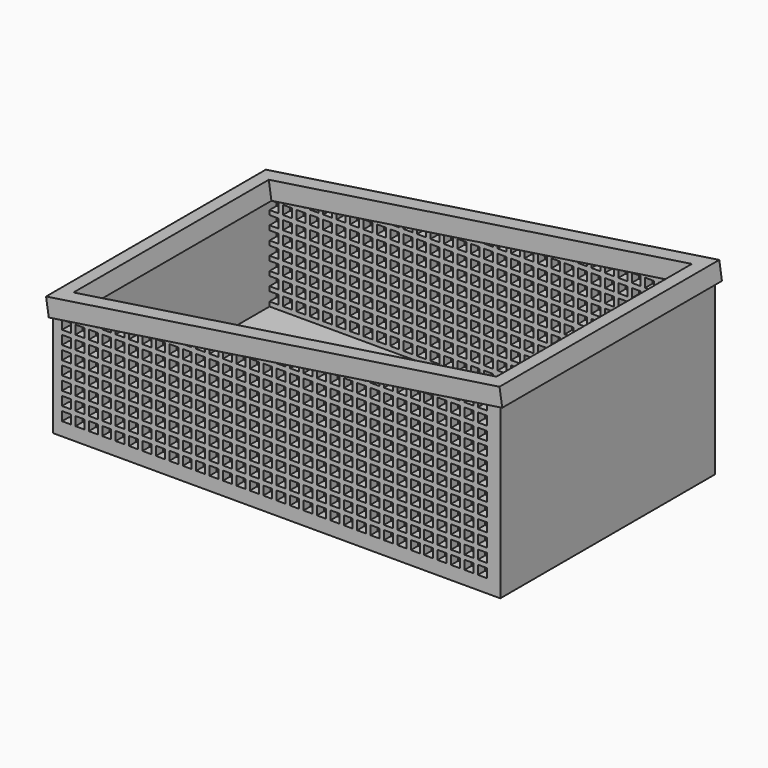
from build123d import *

# Parameters (mm, degrees)
F0_W     = 1270
F0_H     = 762
F1_DEPTH = 508
F3_W     = 1219.2
F3_H     = 711.2
F4_DEPTH = 482.6
F5_DEPTH = 762
F7_W     = 25.4
F7_H     = 25.4
F8_DEPTH = 762
F6_W     = 1302.1685366681
F6_H     = 779.9605122421
F6_W_2   = 1214.8791912068
F6_H_2   = 693.2394877579
F9_DEPTH = 25.4


with BuildPart() as f1:
    # F0 (on Top) → F1 (new body)
    with BuildSketch(Plane.XY):
        with Locations((-15.1927470725, -190.3446181417)):
            Rectangle(F0_W, F0_H)
    extrude(amount=F1_DEPTH)

    # F3 (on face) → F4 (cut)
    with BuildSketch(Plane.XY.offset(508)):
        with Locations((-15.1927470725, -190.3446181417)):
            Rectangle(F3_W, F3_H)
    extrude(amount=-F4_DEPTH, mode=Mode.SUBTRACT)

    # F2 (on face) → F5 (cut)
    with BuildSketch(Plane.XZ.offset(571.3446181417)):
        Polygon((-650.1927470725, 508), (-650.1927470725, 317.5), (619.8072529275, 508), align=None)
    extrude(amount=-F5_DEPTH, mode=Mode.SUBTRACT)

    # F7 (on face) → F8 (cut)
    with BuildSketch(Plane(origin=(0, 190.6553818583, 0), x_dir=(-1, 0, 0), z_dir=(0, 1, 0))):
        with Locations((-569.0072529275, 50.8)):
            Rectangle(F7_W, F7_H)
        with Locations((-569.0072529275, 88.9)):
            Rectangle(F7_W, F7_H)
        with Locations((-569.0072529275, 127)):
            Rectangle(F7_W, F7_H)
        with Locations((-569.0072529275, 165.1)):
            Rectangle(F7_W, F7_H)
        with Locations((-569.0072529275, 203.2)):
            Rectangle(F7_W, F7_H)
        with Locations((-569.0072529275, 241.3)):
            Rectangle(F7_W, F7_H)
        with Locations((-569.0072529275, 279.4)):
            Rectangle(F7_W, F7_H)
        with Locations((-569.0072529275, 317.5)):
            Rectangle(F7_W, F7_H)
        with Locations((-569.0072529275, 355.6)):
            Rectangle(F7_W, F7_H)
        with Locations((-530.9072529275, 50.8)):
            Rectangle(F7_W, F7_H)
        with Locations((-530.9072529275, 88.9)):
            Rectangle(F7_W, F7_H)
        with Locations((-530.9072529275, 127)):
            Rectangle(F7_W, F7_H)
        with Locations((-530.9072529275, 165.1)):
            Rectangle(F7_W, F7_H)
        with Locations((-530.9072529275, 203.2)):
            Rectangle(F7_W, F7_H)
        with Locations((-530.9072529275, 241.3)):
            Rectangle(F7_W, F7_H)
        with Locations((-530.9072529275, 279.4)):
            Rectangle(F7_W, F7_H)
        with Locations((-530.9072529275, 317.5)):
            Rectangle(F7_W, F7_H)
        with Locations((-530.9072529275, 355.6)):
            Rectangle(F7_W, F7_H)
        with Locations((-492.8072529275, 50.8)):
            Rectangle(F7_W, F7_H)
        with Locations((-492.8072529275, 88.9)):
            Rectangle(F7_W, F7_H)
        with Locations((-492.8072529275, 127)):
            Rectangle(F7_W, F7_H)
        with Locations((-492.8072529275, 165.1)):
            Rectangle(F7_W, F7_H)
        with Locations((-492.8072529275, 203.2)):
            Rectangle(F7_W, F7_H)
        with Locations((-492.8072529275, 241.3)):
            Rectangle(F7_W, F7_H)
        with Locations((-492.8072529275, 279.4)):
            Rectangle(F7_W, F7_H)
        with Locations((-492.8072529275, 317.5)):
            Rectangle(F7_W, F7_H)
        with Locations((-492.8072529275, 355.6)):
            Rectangle(F7_W, F7_H)
        with Locations((-454.7072529275, 50.8)):
            Rectangle(F7_W, F7_H)
        with Locations((-454.7072529275, 88.9)):
            Rectangle(F7_W, F7_H)
        with Locations((-454.7072529275, 127)):
            Rectangle(F7_W, F7_H)
        with Locations((-454.7072529275, 165.1)):
            Rectangle(F7_W, F7_H)
        with Locations((-454.7072529275, 203.2)):
            Rectangle(F7_W, F7_H)
        with Locations((-454.7072529275, 241.3)):
            Rectangle(F7_W, F7_H)
        with Locations((-454.7072529275, 279.4)):
            Rectangle(F7_W, F7_H)
        with Locations((-454.7072529275, 317.5)):
            Rectangle(F7_W, F7_H)
        with Locations((-454.7072529275, 355.6)):
            Rectangle(F7_W, F7_H)
        with Locations((-416.6072529275, 50.8)):
            Rectangle(F7_W, F7_H)
        with Locations((-416.6072529275, 88.9)):
            Rectangle(F7_W, F7_H)
        with Locations((-416.6072529275, 127)):
            Rectangle(F7_W, F7_H)
        with Locations((-416.6072529275, 165.1)):
            Rectangle(F7_W, F7_H)
        with Locations((-416.6072529275, 203.2)):
            Rectangle(F7_W, F7_H)
        with Locations((-416.6072529275, 241.3)):
            Rectangle(F7_W, F7_H)
        with Locations((-416.6072529275, 279.4)):
            Rectangle(F7_W, F7_H)
        with Locations((-416.6072529275, 317.5)):
            Rectangle(F7_W, F7_H)
        with Locations((-416.6072529275, 355.6)):
            Rectangle(F7_W, F7_H)
        with Locations((-378.5072529275, 50.8)):
            Rectangle(F7_W, F7_H)
        with Locations((-378.5072529275, 88.9)):
            Rectangle(F7_W, F7_H)
        with Locations((-378.5072529275, 127)):
            Rectangle(F7_W, F7_H)
        with Locations((-378.5072529275, 165.1)):
            Rectangle(F7_W, F7_H)
        with Locations((-378.5072529275, 203.2)):
            Rectangle(F7_W, F7_H)
        with Locations((-378.5072529275, 241.3)):
            Rectangle(F7_W, F7_H)
        with Locations((-378.5072529275, 279.4)):
            Rectangle(F7_W, F7_H)
        with Locations((-378.5072529275, 317.5)):
            Rectangle(F7_W, F7_H)
        with Locations((-378.5072529275, 355.6)):
            Rectangle(F7_W, F7_H)
        with Locations((-340.4072529275, 50.8)):
            Rectangle(F7_W, F7_H)
        with Locations((-340.4072529275, 88.9)):
            Rectangle(F7_W, F7_H)
        with Locations((-340.4072529275, 127)):
            Rectangle(F7_W, F7_H)
        with Locations((-340.4072529275, 165.1)):
            Rectangle(F7_W, F7_H)
        with Locations((-340.4072529275, 203.2)):
            Rectangle(F7_W, F7_H)
        with Locations((-340.4072529275, 241.3)):
            Rectangle(F7_W, F7_H)
        with Locations((-340.4072529275, 279.4)):
            Rectangle(F7_W, F7_H)
        with Locations((-340.4072529275, 317.5)):
            Rectangle(F7_W, F7_H)
        with Locations((-340.4072529275, 355.6)):
            Rectangle(F7_W, F7_H)
        with Locations((-302.3072529275, 50.8)):
            Rectangle(F7_W, F7_H)
        with Locations((-302.3072529275, 88.9)):
            Rectangle(F7_W, F7_H)
        with Locations((-302.3072529275, 127)):
            Rectangle(F7_W, F7_H)
        with Locations((-302.3072529275, 165.1)):
            Rectangle(F7_W, F7_H)
        with Locations((-302.3072529275, 203.2)):
            Rectangle(F7_W, F7_H)
        with Locations((-302.3072529275, 241.3)):
            Rectangle(F7_W, F7_H)
        with Locations((-302.3072529275, 279.4)):
            Rectangle(F7_W, F7_H)
        with Locations((-302.3072529275, 317.5)):
            Rectangle(F7_W, F7_H)
        with Locations((-302.3072529275, 355.6)):
            Rectangle(F7_W, F7_H)
        with Locations((-264.2072529275, 50.8)):
            Rectangle(F7_W, F7_H)
        with Locations((-264.2072529275, 88.9)):
            Rectangle(F7_W, F7_H)
        with Locations((-264.2072529275, 127)):
            Rectangle(F7_W, F7_H)
        with Locations((-264.2072529275, 165.1)):
            Rectangle(F7_W, F7_H)
        with Locations((-264.2072529275, 203.2)):
            Rectangle(F7_W, F7_H)
        with Locations((-264.2072529275, 241.3)):
            Rectangle(F7_W, F7_H)
        with Locations((-264.2072529275, 279.4)):
            Rectangle(F7_W, F7_H)
        with Locations((-264.2072529275, 317.5)):
            Rectangle(F7_W, F7_H)
        with Locations((-264.2072529275, 355.6)):
            Rectangle(F7_W, F7_H)
        with Locations((-226.1072529275, 50.8)):
            Rectangle(F7_W, F7_H)
        with Locations((-226.1072529275, 88.9)):
            Rectangle(F7_W, F7_H)
        with Locations((-226.1072529275, 127)):
            Rectangle(F7_W, F7_H)
        with Locations((-226.1072529275, 165.1)):
            Rectangle(F7_W, F7_H)
        with Locations((-226.1072529275, 203.2)):
            Rectangle(F7_W, F7_H)
        with Locations((-226.1072529275, 241.3)):
            Rectangle(F7_W, F7_H)
        with Locations((-226.1072529275, 279.4)):
            Rectangle(F7_W, F7_H)
        with Locations((-226.1072529275, 317.5)):
            Rectangle(F7_W, F7_H)
        with Locations((-226.1072529275, 355.6)):
            Rectangle(F7_W, F7_H)
        with Locations((-188.0072529275, 50.8)):
            Rectangle(F7_W, F7_H)
        with Locations((-188.0072529275, 88.9)):
            Rectangle(F7_W, F7_H)
        with Locations((-188.0072529275, 127)):
            Rectangle(F7_W, F7_H)
        with Locations((-188.0072529275, 165.1)):
            Rectangle(F7_W, F7_H)
        with Locations((-188.0072529275, 203.2)):
            Rectangle(F7_W, F7_H)
        with Locations((-188.0072529275, 241.3)):
            Rectangle(F7_W, F7_H)
        with Locations((-188.0072529275, 279.4)):
            Rectangle(F7_W, F7_H)
        with Locations((-188.0072529275, 317.5)):
            Rectangle(F7_W, F7_H)
        with Locations((-188.0072529275, 355.6)):
            Rectangle(F7_W, F7_H)
        with Locations((-149.9072529275, 50.8)):
            Rectangle(F7_W, F7_H)
        with Locations((-149.9072529275, 88.9)):
            Rectangle(F7_W, F7_H)
        with Locations((-149.9072529275, 127)):
            Rectangle(F7_W, F7_H)
        with Locations((-149.9072529275, 165.1)):
            Rectangle(F7_W, F7_H)
        with Locations((-149.9072529275, 203.2)):
            Rectangle(F7_W, F7_H)
        with Locations((-149.9072529275, 241.3)):
            Rectangle(F7_W, F7_H)
        with Locations((-149.9072529275, 279.4)):
            Rectangle(F7_W, F7_H)
        with Locations((-149.9072529275, 317.5)):
            Rectangle(F7_W, F7_H)
        with Locations((-149.9072529275, 355.6)):
            Rectangle(F7_W, F7_H)
        with Locations((-111.8072529275, 50.8)):
            Rectangle(F7_W, F7_H)
        with Locations((-111.8072529275, 88.9)):
            Rectangle(F7_W, F7_H)
        with Locations((-111.8072529275, 127)):
            Rectangle(F7_W, F7_H)
        with Locations((-111.8072529275, 165.1)):
            Rectangle(F7_W, F7_H)
        with Locations((-111.8072529275, 203.2)):
            Rectangle(F7_W, F7_H)
        with Locations((-111.8072529275, 241.3)):
            Rectangle(F7_W, F7_H)
        with Locations((-111.8072529275, 279.4)):
            Rectangle(F7_W, F7_H)
        with Locations((-111.8072529275, 317.5)):
            Rectangle(F7_W, F7_H)
        with Locations((-111.8072529275, 355.6)):
            Rectangle(F7_W, F7_H)
        with Locations((-73.7072529275, 50.8)):
            Rectangle(F7_W, F7_H)
        with Locations((-73.7072529275, 88.9)):
            Rectangle(F7_W, F7_H)
        with Locations((-73.7072529275, 127)):
            Rectangle(F7_W, F7_H)
        with Locations((-73.7072529275, 165.1)):
            Rectangle(F7_W, F7_H)
        with Locations((-73.7072529275, 203.2)):
            Rectangle(F7_W, F7_H)
        with Locations((-73.7072529275, 241.3)):
            Rectangle(F7_W, F7_H)
        with Locations((-73.7072529275, 279.4)):
            Rectangle(F7_W, F7_H)
        with Locations((-73.7072529275, 317.5)):
            Rectangle(F7_W, F7_H)
        with Locations((-73.7072529275, 355.6)):
            Rectangle(F7_W, F7_H)
        with Locations((-35.6072529275, 50.8)):
            Rectangle(F7_W, F7_H)
        with Locations((-35.6072529275, 88.9)):
            Rectangle(F7_W, F7_H)
        with Locations((-35.6072529275, 127)):
            Rectangle(F7_W, F7_H)
        with Locations((-35.6072529275, 165.1)):
            Rectangle(F7_W, F7_H)
        with Locations((-35.6072529275, 203.2)):
            Rectangle(F7_W, F7_H)
        with Locations((-35.6072529275, 241.3)):
            Rectangle(F7_W, F7_H)
        with Locations((-35.6072529275, 279.4)):
            Rectangle(F7_W, F7_H)
        with Locations((-35.6072529275, 317.5)):
            Rectangle(F7_W, F7_H)
        with Locations((-35.6072529275, 355.6)):
            Rectangle(F7_W, F7_H)
        with Locations((2.4927470725, 50.8)):
            Rectangle(F7_W, F7_H)
        with Locations((2.4927470725, 88.9)):
            Rectangle(F7_W, F7_H)
        with Locations((2.4927470725, 127)):
            Rectangle(F7_W, F7_H)
        with Locations((2.4927470725, 165.1)):
            Rectangle(F7_W, F7_H)
        with Locations((2.4927470725, 203.2)):
            Rectangle(F7_W, F7_H)
        with Locations((2.4927470725, 241.3)):
            Rectangle(F7_W, F7_H)
        with Locations((2.4927470725, 279.4)):
            Rectangle(F7_W, F7_H)
        with Locations((2.4927470725, 317.5)):
            Rectangle(F7_W, F7_H)
        with Locations((2.4927470725, 355.6)):
            Rectangle(F7_W, F7_H)
        with Locations((40.5927470725, 50.8)):
            Rectangle(F7_W, F7_H)
        with Locations((40.5927470725, 88.9)):
            Rectangle(F7_W, F7_H)
        with Locations((40.5927470725, 127)):
            Rectangle(F7_W, F7_H)
        with Locations((40.5927470725, 165.1)):
            Rectangle(F7_W, F7_H)
        with Locations((40.5927470725, 203.2)):
            Rectangle(F7_W, F7_H)
        with Locations((40.5927470725, 241.3)):
            Rectangle(F7_W, F7_H)
        with Locations((40.5927470725, 279.4)):
            Rectangle(F7_W, F7_H)
        with Locations((40.5927470725, 317.5)):
            Rectangle(F7_W, F7_H)
        with Locations((40.5927470725, 355.6)):
            Rectangle(F7_W, F7_H)
        with Locations((78.6927470725, 50.8)):
            Rectangle(F7_W, F7_H)
        with Locations((78.6927470725, 88.9)):
            Rectangle(F7_W, F7_H)
        with Locations((78.6927470725, 127)):
            Rectangle(F7_W, F7_H)
        with Locations((78.6927470725, 165.1)):
            Rectangle(F7_W, F7_H)
        with Locations((78.6927470725, 203.2)):
            Rectangle(F7_W, F7_H)
        with Locations((78.6927470725, 241.3)):
            Rectangle(F7_W, F7_H)
        with Locations((78.6927470725, 279.4)):
            Rectangle(F7_W, F7_H)
        with Locations((78.6927470725, 317.5)):
            Rectangle(F7_W, F7_H)
        with Locations((78.6927470725, 355.6)):
            Rectangle(F7_W, F7_H)
        with Locations((116.7927470725, 50.8)):
            Rectangle(F7_W, F7_H)
        with Locations((116.7927470725, 88.9)):
            Rectangle(F7_W, F7_H)
        with Locations((116.7927470725, 127)):
            Rectangle(F7_W, F7_H)
        with Locations((116.7927470725, 165.1)):
            Rectangle(F7_W, F7_H)
        with Locations((116.7927470725, 203.2)):
            Rectangle(F7_W, F7_H)
        with Locations((116.7927470725, 241.3)):
            Rectangle(F7_W, F7_H)
        with Locations((116.7927470725, 279.4)):
            Rectangle(F7_W, F7_H)
        with Locations((116.7927470725, 317.5)):
            Rectangle(F7_W, F7_H)
        with Locations((116.7927470725, 355.6)):
            Rectangle(F7_W, F7_H)
        with Locations((154.8927470725, 50.8)):
            Rectangle(F7_W, F7_H)
        with Locations((154.8927470725, 88.9)):
            Rectangle(F7_W, F7_H)
        with Locations((154.8927470725, 127)):
            Rectangle(F7_W, F7_H)
        with Locations((154.8927470725, 165.1)):
            Rectangle(F7_W, F7_H)
        with Locations((154.8927470725, 203.2)):
            Rectangle(F7_W, F7_H)
        with Locations((154.8927470725, 241.3)):
            Rectangle(F7_W, F7_H)
        with Locations((154.8927470725, 279.4)):
            Rectangle(F7_W, F7_H)
        with Locations((154.8927470725, 317.5)):
            Rectangle(F7_W, F7_H)
        with Locations((154.8927470725, 355.6)):
            Rectangle(F7_W, F7_H)
        with Locations((192.9927470725, 50.8)):
            Rectangle(F7_W, F7_H)
        with Locations((192.9927470725, 88.9)):
            Rectangle(F7_W, F7_H)
        with Locations((192.9927470725, 127)):
            Rectangle(F7_W, F7_H)
        with Locations((192.9927470725, 165.1)):
            Rectangle(F7_W, F7_H)
        with Locations((192.9927470725, 203.2)):
            Rectangle(F7_W, F7_H)
        with Locations((192.9927470725, 241.3)):
            Rectangle(F7_W, F7_H)
        with Locations((192.9927470725, 279.4)):
            Rectangle(F7_W, F7_H)
        with Locations((192.9927470725, 317.5)):
            Rectangle(F7_W, F7_H)
        with Locations((192.9927470725, 355.6)):
            Rectangle(F7_W, F7_H)
        with Locations((231.0927470725, 50.8)):
            Rectangle(F7_W, F7_H)
        with Locations((231.0927470725, 88.9)):
            Rectangle(F7_W, F7_H)
        with Locations((231.0927470725, 127)):
            Rectangle(F7_W, F7_H)
        with Locations((231.0927470725, 165.1)):
            Rectangle(F7_W, F7_H)
        with Locations((231.0927470725, 203.2)):
            Rectangle(F7_W, F7_H)
        with Locations((231.0927470725, 241.3)):
            Rectangle(F7_W, F7_H)
        with Locations((231.0927470725, 279.4)):
            Rectangle(F7_W, F7_H)
        with Locations((231.0927470725, 317.5)):
            Rectangle(F7_W, F7_H)
        with Locations((231.0927470725, 355.6)):
            Rectangle(F7_W, F7_H)
        with Locations((269.1927470725, 50.8)):
            Rectangle(F7_W, F7_H)
        with Locations((269.1927470725, 88.9)):
            Rectangle(F7_W, F7_H)
        with Locations((269.1927470725, 127)):
            Rectangle(F7_W, F7_H)
        with Locations((269.1927470725, 165.1)):
            Rectangle(F7_W, F7_H)
        with Locations((269.1927470725, 203.2)):
            Rectangle(F7_W, F7_H)
        with Locations((269.1927470725, 241.3)):
            Rectangle(F7_W, F7_H)
        with Locations((269.1927470725, 279.4)):
            Rectangle(F7_W, F7_H)
        with Locations((269.1927470725, 317.5)):
            Rectangle(F7_W, F7_H)
        with Locations((269.1927470725, 355.6)):
            Rectangle(F7_W, F7_H)
        with Locations((307.2927470725, 50.8)):
            Rectangle(F7_W, F7_H)
        with Locations((307.2927470725, 88.9)):
            Rectangle(F7_W, F7_H)
        with Locations((307.2927470725, 127)):
            Rectangle(F7_W, F7_H)
        with Locations((307.2927470725, 165.1)):
            Rectangle(F7_W, F7_H)
        with Locations((307.2927470725, 203.2)):
            Rectangle(F7_W, F7_H)
        with Locations((307.2927470725, 241.3)):
            Rectangle(F7_W, F7_H)
        with Locations((307.2927470725, 279.4)):
            Rectangle(F7_W, F7_H)
        with Locations((307.2927470725, 317.5)):
            Rectangle(F7_W, F7_H)
        with Locations((307.2927470725, 355.6)):
            Rectangle(F7_W, F7_H)
        with Locations((-569.0072529275, 393.7)):
            Rectangle(F7_W, F7_H)
        with Locations((-530.9072529275, 393.7)):
            Rectangle(F7_W, F7_H)
        with Locations((-492.8072529275, 393.7)):
            Rectangle(F7_W, F7_H)
        with Locations((-454.7072529275, 393.7)):
            Rectangle(F7_W, F7_H)
        with Locations((-416.6072529275, 393.7)):
            Rectangle(F7_W, F7_H)
        with Locations((-378.5072529275, 393.7)):
            Rectangle(F7_W, F7_H)
        with Locations((-340.4072529275, 393.7)):
            Rectangle(F7_W, F7_H)
        with Locations((-302.3072529275, 393.7)):
            Rectangle(F7_W, F7_H)
        with Locations((-264.2072529275, 393.7)):
            Rectangle(F7_W, F7_H)
        with Locations((-226.1072529275, 393.7)):
            Rectangle(F7_W, F7_H)
        with Locations((-188.0072529275, 393.7)):
            Rectangle(F7_W, F7_H)
        with Locations((-149.9072529275, 393.7)):
            Rectangle(F7_W, F7_H)
        with Locations((-111.8072529275, 393.7)):
            Rectangle(F7_W, F7_H)
        with Locations((-73.7072529275, 393.7)):
            Rectangle(F7_W, F7_H)
        with Locations((-35.6072529275, 393.7)):
            Rectangle(F7_W, F7_H)
        with Locations((2.4927470725, 393.7)):
            Rectangle(F7_W, F7_H)
        with Locations((40.5927470725, 393.7)):
            Rectangle(F7_W, F7_H)
        with Locations((78.6927470725, 393.7)):
            Rectangle(F7_W, F7_H)
        with Locations((116.7927470725, 393.7)):
            Rectangle(F7_W, F7_H)
        with Locations((154.8927470725, 393.7)):
            Rectangle(F7_W, F7_H)
        with Locations((192.9927470725, 393.7)):
            Rectangle(F7_W, F7_H)
        with Locations((231.0927470725, 393.7)):
            Rectangle(F7_W, F7_H)
        with Locations((269.1927470725, 393.7)):
            Rectangle(F7_W, F7_H)
        with Locations((307.2927470725, 393.7)):
            Rectangle(F7_W, F7_H)
        with Locations((345.3927470725, 50.8)):
            Rectangle(F7_W, F7_H)
        with Locations((345.3927470725, 88.9)):
            Rectangle(F7_W, F7_H)
        with Locations((345.3927470725, 127)):
            Rectangle(F7_W, F7_H)
        with Locations((345.3927470725, 165.1)):
            Rectangle(F7_W, F7_H)
        with Locations((345.3927470725, 203.2)):
            Rectangle(F7_W, F7_H)
        with Locations((345.3927470725, 241.3)):
            Rectangle(F7_W, F7_H)
        with Locations((345.3927470725, 279.4)):
            Rectangle(F7_W, F7_H)
        with Locations((345.3927470725, 317.5)):
            Rectangle(F7_W, F7_H)
        with Locations((345.3927470725, 355.6)):
            Rectangle(F7_W, F7_H)
        with Locations((345.3927470725, 393.7)):
            Rectangle(F7_W, F7_H)
        with Locations((-569.0072529275, 431.8)):
            Rectangle(F7_W, F7_H)
        with Locations((-569.0072529275, 469.9)):
            Rectangle(F7_W, F7_H)
        with Locations((-530.9072529275, 431.8)):
            Rectangle(F7_W, F7_H)
        with Locations((-530.9072529275, 469.9)):
            Rectangle(F7_W, F7_H)
        with Locations((-492.8072529275, 431.8)):
            Rectangle(F7_W, F7_H)
        with Locations((-492.8072529275, 469.9)):
            Rectangle(F7_W, F7_H)
        with Locations((-454.7072529275, 431.8)):
            Rectangle(F7_W, F7_H)
        with Locations((-454.7072529275, 469.9)):
            Rectangle(F7_W, F7_H)
        with Locations((-416.6072529275, 431.8)):
            Rectangle(F7_W, F7_H)
        with Locations((-416.6072529275, 469.9)):
            Rectangle(F7_W, F7_H)
        with Locations((-378.5072529275, 431.8)):
            Rectangle(F7_W, F7_H)
        with Locations((-378.5072529275, 469.9)):
            Rectangle(F7_W, F7_H)
        with Locations((-340.4072529275, 431.8)):
            Rectangle(F7_W, F7_H)
        with Locations((-340.4072529275, 469.9)):
            Rectangle(F7_W, F7_H)
        with Locations((-302.3072529275, 431.8)):
            Rectangle(F7_W, F7_H)
        with Locations((-302.3072529275, 469.9)):
            Rectangle(F7_W, F7_H)
        with Locations((-264.2072529275, 431.8)):
            Rectangle(F7_W, F7_H)
        with Locations((-264.2072529275, 469.9)):
            Rectangle(F7_W, F7_H)
        with Locations((-226.1072529275, 431.8)):
            Rectangle(F7_W, F7_H)
        with Locations((-226.1072529275, 469.9)):
            Rectangle(F7_W, F7_H)
        with Locations((-188.0072529275, 431.8)):
            Rectangle(F7_W, F7_H)
        with Locations((-188.0072529275, 469.9)):
            Rectangle(F7_W, F7_H)
        with Locations((-149.9072529275, 431.8)):
            Rectangle(F7_W, F7_H)
        with Locations((-149.9072529275, 469.9)):
            Rectangle(F7_W, F7_H)
        with Locations((-111.8072529275, 431.8)):
            Rectangle(F7_W, F7_H)
        with Locations((-111.8072529275, 469.9)):
            Rectangle(F7_W, F7_H)
        with Locations((-73.7072529275, 431.8)):
            Rectangle(F7_W, F7_H)
        with Locations((-73.7072529275, 469.9)):
            Rectangle(F7_W, F7_H)
        with Locations((-35.6072529275, 431.8)):
            Rectangle(F7_W, F7_H)
        with Locations((-35.6072529275, 469.9)):
            Rectangle(F7_W, F7_H)
        with Locations((2.4927470725, 431.8)):
            Rectangle(F7_W, F7_H)
        with Locations((2.4927470725, 469.9)):
            Rectangle(F7_W, F7_H)
        with Locations((40.5927470725, 431.8)):
            Rectangle(F7_W, F7_H)
        with Locations((40.5927470725, 469.9)):
            Rectangle(F7_W, F7_H)
        with Locations((78.6927470725, 431.8)):
            Rectangle(F7_W, F7_H)
        with Locations((78.6927470725, 469.9)):
            Rectangle(F7_W, F7_H)
        with Locations((116.7927470725, 431.8)):
            Rectangle(F7_W, F7_H)
        with Locations((116.7927470725, 469.9)):
            Rectangle(F7_W, F7_H)
        with Locations((154.8927470725, 431.8)):
            Rectangle(F7_W, F7_H)
        with Locations((154.8927470725, 469.9)):
            Rectangle(F7_W, F7_H)
        with Locations((192.9927470725, 431.8)):
            Rectangle(F7_W, F7_H)
        with Locations((192.9927470725, 469.9)):
            Rectangle(F7_W, F7_H)
        with Locations((231.0927470725, 431.8)):
            Rectangle(F7_W, F7_H)
        with Locations((231.0927470725, 469.9)):
            Rectangle(F7_W, F7_H)
        with Locations((269.1927470725, 431.8)):
            Rectangle(F7_W, F7_H)
        with Locations((269.1927470725, 469.9)):
            Rectangle(F7_W, F7_H)
        with Locations((307.2927470725, 431.8)):
            Rectangle(F7_W, F7_H)
        with Locations((307.2927470725, 469.9)):
            Rectangle(F7_W, F7_H)
        with Locations((345.3927470725, 431.8)):
            Rectangle(F7_W, F7_H)
        with Locations((345.3927470725, 469.9)):
            Rectangle(F7_W, F7_H)
        with Locations((383.4927470725, 50.8)):
            Rectangle(F7_W, F7_H)
        with Locations((383.4927470725, 88.9)):
            Rectangle(F7_W, F7_H)
        with Locations((383.4927470725, 127)):
            Rectangle(F7_W, F7_H)
        with Locations((383.4927470725, 165.1)):
            Rectangle(F7_W, F7_H)
        with Locations((383.4927470725, 203.2)):
            Rectangle(F7_W, F7_H)
        with Locations((383.4927470725, 241.3)):
            Rectangle(F7_W, F7_H)
        with Locations((383.4927470725, 279.4)):
            Rectangle(F7_W, F7_H)
        with Locations((383.4927470725, 317.5)):
            Rectangle(F7_W, F7_H)
        with Locations((383.4927470725, 355.6)):
            Rectangle(F7_W, F7_H)
        with Locations((383.4927470725, 393.7)):
            Rectangle(F7_W, F7_H)
        with Locations((383.4927470725, 431.8)):
            Rectangle(F7_W, F7_H)
        with Locations((383.4927470725, 469.9)):
            Rectangle(F7_W, F7_H)
        with Locations((421.5927470725, 50.8)):
            Rectangle(F7_W, F7_H)
        with Locations((421.5927470725, 88.9)):
            Rectangle(F7_W, F7_H)
        with Locations((421.5927470725, 127)):
            Rectangle(F7_W, F7_H)
        with Locations((421.5927470725, 165.1)):
            Rectangle(F7_W, F7_H)
        with Locations((421.5927470725, 203.2)):
            Rectangle(F7_W, F7_H)
        with Locations((421.5927470725, 241.3)):
            Rectangle(F7_W, F7_H)
        with Locations((421.5927470725, 279.4)):
            Rectangle(F7_W, F7_H)
        with Locations((421.5927470725, 317.5)):
            Rectangle(F7_W, F7_H)
        with Locations((421.5927470725, 355.6)):
            Rectangle(F7_W, F7_H)
        with Locations((421.5927470725, 393.7)):
            Rectangle(F7_W, F7_H)
        with Locations((421.5927470725, 431.8)):
            Rectangle(F7_W, F7_H)
        with Locations((421.5927470725, 469.9)):
            Rectangle(F7_W, F7_H)
        with Locations((459.6927470725, 50.8)):
            Rectangle(F7_W, F7_H)
        with Locations((459.6927470725, 88.9)):
            Rectangle(F7_W, F7_H)
        with Locations((459.6927470725, 127)):
            Rectangle(F7_W, F7_H)
        with Locations((459.6927470725, 165.1)):
            Rectangle(F7_W, F7_H)
        with Locations((459.6927470725, 203.2)):
            Rectangle(F7_W, F7_H)
        with Locations((459.6927470725, 241.3)):
            Rectangle(F7_W, F7_H)
        with Locations((459.6927470725, 279.4)):
            Rectangle(F7_W, F7_H)
        with Locations((459.6927470725, 317.5)):
            Rectangle(F7_W, F7_H)
        with Locations((459.6927470725, 355.6)):
            Rectangle(F7_W, F7_H)
        with Locations((459.6927470725, 393.7)):
            Rectangle(F7_W, F7_H)
        with Locations((459.6927470725, 431.8)):
            Rectangle(F7_W, F7_H)
        with Locations((459.6927470725, 469.9)):
            Rectangle(F7_W, F7_H)
        with Locations((497.7927470725, 50.8)):
            Rectangle(F7_W, F7_H)
        with Locations((497.7927470725, 88.9)):
            Rectangle(F7_W, F7_H)
        with Locations((497.7927470725, 127)):
            Rectangle(F7_W, F7_H)
        with Locations((497.7927470725, 165.1)):
            Rectangle(F7_W, F7_H)
        with Locations((497.7927470725, 203.2)):
            Rectangle(F7_W, F7_H)
        with Locations((497.7927470725, 241.3)):
            Rectangle(F7_W, F7_H)
        with Locations((497.7927470725, 279.4)):
            Rectangle(F7_W, F7_H)
        with Locations((497.7927470725, 317.5)):
            Rectangle(F7_W, F7_H)
        with Locations((497.7927470725, 355.6)):
            Rectangle(F7_W, F7_H)
        with Locations((497.7927470725, 393.7)):
            Rectangle(F7_W, F7_H)
        with Locations((497.7927470725, 431.8)):
            Rectangle(F7_W, F7_H)
        with Locations((497.7927470725, 469.9)):
            Rectangle(F7_W, F7_H)
        with Locations((535.8927470725, 50.8)):
            Rectangle(F7_W, F7_H)
        with Locations((535.8927470725, 88.9)):
            Rectangle(F7_W, F7_H)
        with Locations((535.8927470725, 127)):
            Rectangle(F7_W, F7_H)
        with Locations((535.8927470725, 165.1)):
            Rectangle(F7_W, F7_H)
        with Locations((535.8927470725, 203.2)):
            Rectangle(F7_W, F7_H)
        with Locations((535.8927470725, 241.3)):
            Rectangle(F7_W, F7_H)
        with Locations((535.8927470725, 279.4)):
            Rectangle(F7_W, F7_H)
        with Locations((535.8927470725, 317.5)):
            Rectangle(F7_W, F7_H)
        with Locations((535.8927470725, 355.6)):
            Rectangle(F7_W, F7_H)
        with Locations((535.8927470725, 393.7)):
            Rectangle(F7_W, F7_H)
        with Locations((535.8927470725, 431.8)):
            Rectangle(F7_W, F7_H)
        with Locations((535.8927470725, 469.9)):
            Rectangle(F7_W, F7_H)
        with Locations((573.9927470725, 50.8)):
            Rectangle(F7_W, F7_H)
        with Locations((573.9927470725, 88.9)):
            Rectangle(F7_W, F7_H)
        with Locations((573.9927470725, 127)):
            Rectangle(F7_W, F7_H)
        with Locations((573.9927470725, 165.1)):
            Rectangle(F7_W, F7_H)
        with Locations((573.9927470725, 203.2)):
            Rectangle(F7_W, F7_H)
        with Locations((573.9927470725, 241.3)):
            Rectangle(F7_W, F7_H)
        with Locations((573.9927470725, 279.4)):
            Rectangle(F7_W, F7_H)
        with Locations((573.9927470725, 317.5)):
            Rectangle(F7_W, F7_H)
        with Locations((573.9927470725, 355.6)):
            Rectangle(F7_W, F7_H)
        with Locations((573.9927470725, 393.7)):
            Rectangle(F7_W, F7_H)
        with Locations((573.9927470725, 431.8)):
            Rectangle(F7_W, F7_H)
        with Locations((573.9927470725, 469.9)):
            Rectangle(F7_W, F7_H)
        with Locations((612.0927470725, 50.8)):
            Rectangle(F7_W, F7_H)
        with Locations((612.0927470725, 88.9)):
            Rectangle(F7_W, F7_H)
        with Locations((612.0927470725, 127)):
            Rectangle(F7_W, F7_H)
        with Locations((612.0927470725, 165.1)):
            Rectangle(F7_W, F7_H)
        with Locations((612.0927470725, 203.2)):
            Rectangle(F7_W, F7_H)
        with Locations((612.0927470725, 241.3)):
            Rectangle(F7_W, F7_H)
        with Locations((612.0927470725, 279.4)):
            Rectangle(F7_W, F7_H)
        with Locations((612.0927470725, 317.5)):
            Rectangle(F7_W, F7_H)
        with Locations((612.0927470725, 355.6)):
            Rectangle(F7_W, F7_H)
        with Locations((612.0927470725, 393.7)):
            Rectangle(F7_W, F7_H)
        with Locations((612.0927470725, 431.8)):
            Rectangle(F7_W, F7_H)
        with Locations((612.0927470725, 469.9)):
            Rectangle(F7_W, F7_H)
    extrude(amount=-F8_DEPTH, mode=Mode.SUBTRACT)

    # F6 (on face) → F9 (join, symmetric)
    with BuildSketch(Plane(origin=(-60.8844369771, 0, 405.8962465143), x_dir=(0.9889363529, 0, 0.1483404529), z_dir=(-0.1483404529, 0, 0.9889363529))):
        with Locations((46.2028620671, -190.3446181417)):
            Rectangle(F6_W, F6_H)
        with Locations((46.2028620671, -190.3446181417)):
            Rectangle(F6_W_2, F6_H_2, mode=Mode.SUBTRACT)
    extrude(amount=F9_DEPTH, both=True)


solid = f1.part
